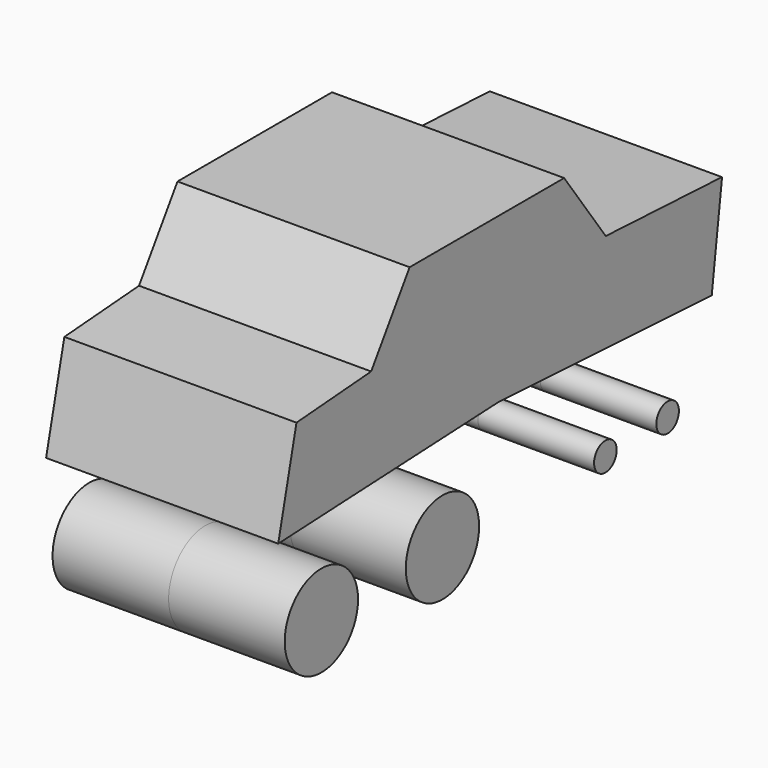
from build123d import *

# Parameters (mm, degrees)
F1_DEPTH = 25.4
F0_R     = 10.0305561335
F0_R_2   = 3.0951686204
F3_DEPTH = 25.4
F2_R     = 10.0305561335
F2_R_2   = 3.0951686204


with BuildPart() as f1:
    # F0 (on Right) → F1 (new body)
    with BuildSketch(Plane.YZ):
        Polygon((-55.0975427032, 28.3502675593), (-60.0938091379, 7.062059809), (0, 9.8499162998), (58.4986023605, 6.6740531474), (61.2806901336, 28.0596334487), (61.2806901336, 28.3502675593), (29.5018939694, 29.9033019692), (18.1195573523, 45.7114391029), (-24.1487864405, 45.7114391029), (-34.6697121859, 29.9033019692), align=None)
    extrude(amount=-F1_DEPTH)

    # F2 (on Right) → F3 (join)
    with BuildSketch(Plane.YZ):
        Polygon((-60.0938091379, 7.062059809), (0, 9.8499162998), (58.4986023605, 6.6740531474), (61.2806901336, 28.0596334487), (61.2806901336, 28.3502675593), (29.5018939694, 29.9033019692), (18.1195573523, 45.7114391029), (-24.1487864405, 45.7114391029), (-34.6697121859, 29.9033019692), (-55.0975427032, 28.3502675593), align=None)
    extrude(amount=F3_DEPTH)


with BuildPart() as f1b:
    # F0 (on Right) → F1, piece 2 (new body)
    with BuildSketch(Plane.YZ):
        with Locations((-48.2845641673, -12.5354165211)):
            Circle(F0_R)
    extrude(amount=-F1_DEPTH)


with BuildPart() as f1c:
    # F0 (on Right) → F1, piece 3 (new body)
    with BuildSketch(Plane.YZ):
        with Locations((-15.1663050056, -11.9163831696)):
            Circle(F0_R)
    extrude(amount=-F1_DEPTH)


with BuildPart() as f1d:
    # F0 (on Right) → F1, piece 4 (new body)
    with BuildSketch(Plane.YZ):
        with Locations((46.4274659753, -11.9163831696)):
            Circle(F0_R_2)
    extrude(amount=-F1_DEPTH)


with BuildPart() as f1e:
    # F0 (on Right) → F1, piece 5 (new body)
    with BuildSketch(Plane.YZ):
        with Locations((29.4040646404, -12.5354165211)):
            Circle(F0_R_2)
    extrude(amount=-F1_DEPTH)


with BuildPart() as f3:
    # F2 (on Right) → F3, piece 2 (new body)
    with BuildSketch(Plane.YZ):
        with Locations((-48.2845641673, -12.5354165211)):
            Circle(F2_R)
    extrude(amount=F3_DEPTH)


with BuildPart() as f3b:
    # F2 (on Right) → F3, piece 3 (new body)
    with BuildSketch(Plane.YZ):
        with Locations((-15.1663050056, -11.9163831696)):
            Circle(F2_R)
    extrude(amount=F3_DEPTH)


with BuildPart() as f3c:
    # F2 (on Right) → F3, piece 4 (new body)
    with BuildSketch(Plane.YZ):
        with Locations((46.4274659753, -11.9163831696)):
            Circle(F2_R_2)
    extrude(amount=F3_DEPTH)


with BuildPart() as f3d:
    # F2 (on Right) → F3, piece 5 (new body)
    with BuildSketch(Plane.YZ):
        with Locations((29.4040646404, -12.5354165211)):
            Circle(F2_R_2)
    extrude(amount=F3_DEPTH)


solid = Compound([f1.part, f1b.part, f1c.part, f1d.part, f1e.part, f3.part, f3b.part, f3c.part, f3d.part])
